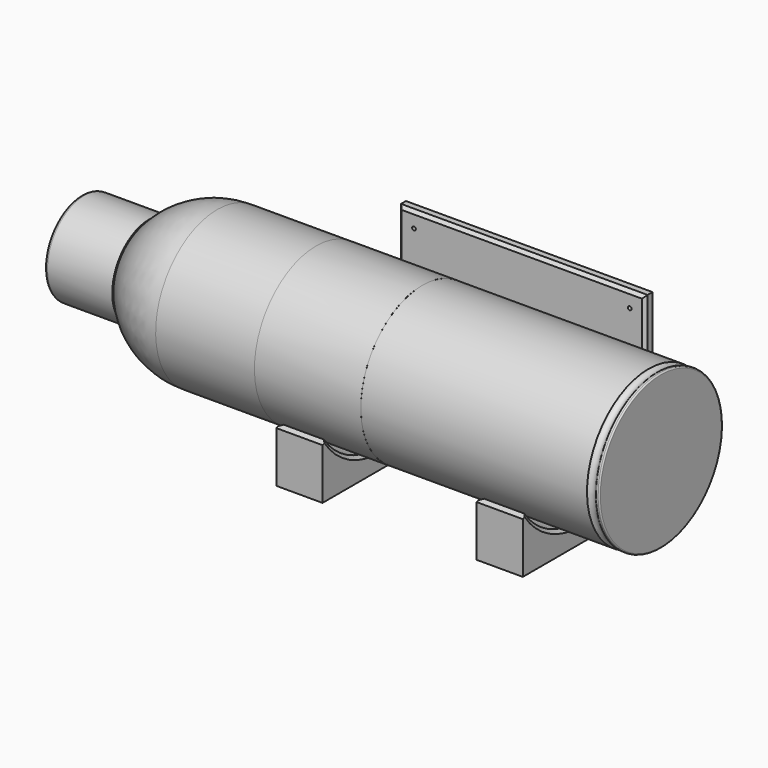
from build123d import *

# Parameters (mm, degrees)
F1_DEPTH     = 50.8
F2_T1_DEPTH  = 124.1425594427
F3_W         = 63.5
F3_H         = 53.3753879368
F4_DEPTH     = 25.4
F5_T1_DEPTH  = 63.5
F5_T3_DEPTH  = 108.1320747894
F5_T5_DEPTH  = 38.570501885
F5_T10_ANGLE = 111.4913949057
F5_T15_ANGLE = 111.4913949057
F5_T18_ANGLE = 150.4795795225
F5_T20_ANGLE = 150.4795795225
F5_T25_DEPTH = 64.906372973
F5_T29_ANGLE = 111.4913949057
F5_T36_ANGLE = 111.4913949057
F5_T40_DEPTH = 64.906372973
F6_R         = 0.762
F7_DEPTH     = 3.81
F10_W        = 5.08
F10_H        = 15.875
F14_R        = 2.54
F19_R        = 0.508
F20_R        = 1.3252507726
F21_DEPTH    = 25.4
F22_W        = 43.8366280696
F22_H        = 31.7754


# Not quite as in the source:
# - a fillet or chamfer that OpenCascade refuses, or shapes differently, is made with other operations: its cross-section is extruded or revolved along the edge and cut away or added
# - a pattern or mirror of a feature is missing from the dataset's text; its kind, count and spacing are read off the source's solid


with BuildPart() as f1:
    # F0 (on Right) → F1 (new body, symmetric)
    with BuildSketch(Plane.YZ):
        with BuildLine():
            Line((33.401, 35.3044644903), (33.401, 0))
            ThreePointArc((33.401, 0), (7.9787555162, -32.4340293737), (-29.58910577, -15.4955355097))
            Line((-29.58910577, -15.4955355097), (-29.58910577, -40.8955355097))
            Line((-29.58910577, -40.8955355097), (37.211, -40.8955355097))
            Line((37.211, -40.8955355097), (37.211, 35.3044644903))
            Line((37.211, 35.3044644903), (33.401, 35.3044644903))
        make_face()
    extrude(amount=F1_DEPTH, both=True)

    # F2: chamfer of 5.08 on 1 edges, made by hand

    # F2_s2 → F2_t1 (cut)
    with BuildSketch(Plane.YZ.offset(-62.0712797213)):
        with BuildLine():
            Line((-29.7828322597, -19.9998833533), (-27.1236395633, -19.1581562557))
            Line((-27.1236395633, -19.1581562557), (-27.0405449137, -19.0996939669))
            ThreePointArc((-27.0405449137, -19.0996939669), (-28.414686405, -17.3624778434), (-29.4991008855, -15.4484008009))
            Line((-29.4991008855, -15.4484008009), (-29.69070577, -15.4955355097))
            ThreePointArc((-29.69070577, -15.4955355097), (-29.69070577, -17.7477094315), (-29.8844322597, -19.9998833533))
            Line((-29.8844322597, -19.9998833533), (-29.7828322597, -19.9998833533))
        make_face()
    extrude(amount=F2_T1_DEPTH, mode=Mode.SUBTRACT)

    # F3 (on face) → F4 (cut)
    with BuildSketch(Plane(origin=(0, 0, -40.8955355097), x_dir=(1, 0, 0), z_dir=(0, 0, -1))):
        with Locations((0, 2.9014118016)):
            Rectangle(F3_W, F3_H)
    extrude(amount=-F4_DEPTH, mode=Mode.SUBTRACT)

    # F5: chamfer of 1.27 on 8 edges, made by hand

    # F5_s2 → F5_t1 (cut)
    with BuildSketch(Plane.YZ.offset(-31.75)):
        with BuildLine():
            Line((24.1384696333, -23.0859499429), (23.7862821668, -23.9637427164))
            Line((23.7862821668, -23.9637427164), (23.7862821668, -23.4486584196))
            ThreePointArc((23.7862821668, -23.4486584196), (23.9794328881, -23.2510988852), (24.1384696333, -23.0859499429))
        make_face()
    extrude(amount=F5_T1_DEPTH, mode=Mode.SUBTRACT)

    # F5_s4 → F5_t3 (cut)
    with BuildSketch(Plane.YZ.offset(-54.0660373947)):
        Polygon((34.671, 35.3044644903), (33.401, 34.0344644903), (33.401, 35.3044644903), align=None)
    extrude(amount=F5_T3_DEPTH, mode=Mode.SUBTRACT)

    # F5_s6 → F5_t5 (cut)
    with BuildSketch(Plane.XY):
        Polygon((-50.8, 34.671), (-49.53, 33.401), (-50.8, 33.401), align=None)
        Polygon((50.8, 34.671), (49.53, 33.401), (50.8, 33.401), align=None)
    extrude(amount=F5_T5_DEPTH, mode=Mode.SUBTRACT)


with BuildPart() as f5_tool8:
    # F5_s9 → F5_t10 (revolve)
    with BuildSketch(Plane(origin=(0, 0, 0), x_dir=(1, 0, 0), z_dir=(0, -0.4927798926, 0.8701539964))):
        Polygon((-33.02, -33.401), (-31.75, -34.671), (-31.75, -33.401), align=None)
    revolve(axis=Axis((-31.75, 0, 0), (1, 0, 0)), revolution_arc=F5_T10_ANGLE)

    split(bisect_by=Plane.XZ.offset(-23.7862821668), keep=Keep.TOP)


with BuildPart() as f1_1:
    add(f1.part)

    # F5_t7: cut F5_tool8
    add(f5_tool8.part, mode=Mode.SUBTRACT)


with BuildPart() as f5_tool13:
    # F5_s14 → F5_t15 (revolve)
    with BuildSketch(Plane(origin=(0, 0, 0), x_dir=(1, 0, 0), z_dir=(0, -0.4927798926, 0.8701539964))):
        Polygon((33.02, -33.401), (31.75, -34.671), (31.75, -33.401), align=None)
    revolve(axis=Axis((31.75, 0, 0), (1, 0, 0)), revolution_arc=F5_T15_ANGLE)

    split(bisect_by=Plane.XZ.offset(-23.7862821668), keep=Keep.TOP)


with BuildPart() as f1_2:
    add(f1_1.part)

    # F5_t12: cut F5_tool13
    add(f5_tool13.part, mode=Mode.SUBTRACT)

    # F5_s17 → F5_t18 (revolve, cut)
    with BuildSketch(Plane.XY):
        Polygon((50.8, 34.671), (49.53, 33.401), (50.8, 33.401), align=None)
    revolve(axis=Axis((50.8, 0, 0), (-1, 0, 0)), revolution_arc=F5_T18_ANGLE, mode=Mode.SUBTRACT)

    # F5_s19 → F5_t20 (revolve, cut)
    with BuildSketch(Plane.XY):
        Polygon((-50.8, 34.671), (-49.53, 33.401), (-50.8, 33.401), align=None)
    revolve(axis=Axis((-50.8, 0, 0), (-1, 0, 0)), revolution_arc=F5_T20_ANGLE, mode=Mode.SUBTRACT)


with BuildPart() as f5_tool23:
    # F5_s24 → F5_t25 (new body)
    with BuildSketch(Plane.YZ.offset(-33.156372973)):
        with BuildLine():
            Line((24.1384696333, -23.0859499429), (23.7862821668, -23.9637427164))
            Line((23.7862821668, -23.9637427164), (23.7862821668, -23.4486584196))
            ThreePointArc((23.7862821668, -23.4486584196), (23.9794328881, -23.2510988852), (24.1384696333, -23.0859499429))
        make_face()
    extrude(amount=F5_T25_DEPTH)

    split(bisect_by=Plane.YZ.offset(-31.75), keep=Keep.BOTTOM)


with BuildPart() as f5_tool27:
    # F5_s28 → F5_t29 (revolve)
    with BuildSketch(Plane(origin=(0, 0, 0), x_dir=(1, 0, 0), z_dir=(0, -0.4927798926, 0.8701539964))):
        Polygon((-33.02, -33.401), (-31.75, -34.671), (-31.75, -33.401), align=None)
    revolve(axis=Axis((-31.75, 0, 0), (1, 0, 0)), revolution_arc=F5_T29_ANGLE)

    split(bisect_by=Plane.XZ.offset(-23.7862821668), keep=Keep.BOTTOM)


with BuildPart() as f5_tool23_1:
    add(f5_tool23.part)

    # F5_t31: intersect F5_tool27
    add(f5_tool27.part, mode=Mode.INTERSECT)


with BuildPart() as f1_3:
    add(f1_2.part)

    # F5_t21: cut F5_tool23
    add(f5_tool23_1.part, mode=Mode.SUBTRACT)


with BuildPart() as f5_tool34:
    # F5_s35 → F5_t36 (revolve)
    with BuildSketch(Plane(origin=(0, 0, 0), x_dir=(1, 0, 0), z_dir=(0, -0.4927798926, 0.8701539964))):
        Polygon((33.02, -33.401), (31.75, -34.671), (31.75, -33.401), align=None)
    revolve(axis=Axis((31.75, 0, 0), (1, 0, 0)), revolution_arc=F5_T36_ANGLE)

    split(bisect_by=Plane.XZ.offset(-23.7862821668), keep=Keep.BOTTOM)


with BuildPart() as f5_tool38:
    # F5_s39 → F5_t40 (new body)
    with BuildSketch(Plane.YZ.offset(-31.75)):
        with BuildLine():
            Line((24.1384696333, -23.0859499429), (23.7862821668, -23.9637427164))
            Line((23.7862821668, -23.9637427164), (23.7862821668, -23.4486584196))
            ThreePointArc((23.7862821668, -23.4486584196), (23.9794328881, -23.2510988852), (24.1384696333, -23.0859499429))
        make_face()
    extrude(amount=F5_T40_DEPTH)

    split(bisect_by=Plane.YZ.offset(31.75), keep=Keep.TOP)


with BuildPart() as f5_tool34_1:
    add(f5_tool34.part)

    # F5_t42: intersect F5_tool38
    add(f5_tool38.part, mode=Mode.INTERSECT)


with BuildPart() as f1_4:
    add(f1_3.part)

    # F5_t32: cut F5_tool34
    add(f5_tool34_1.part, mode=Mode.SUBTRACT)

    # F6 (on face) → F7 (cut, through all)
    with BuildSketch(Plane(origin=(0, 37.211, 0), x_dir=(-1, 0, 0), z_dir=(0, 1, 0))):
        with Locations((-44.45, 28.9544644903)):
            Circle(F6_R)
    f7 = extrude(amount=-F7_DEPTH, mode=Mode.SUBTRACT)

    # F7_copies: F7 across plane
    add(f7.mirror(Plane(origin=(0, 0, 0), x_dir=(0, 0, -1), z_dir=(-1, 0, 0))), mode=Mode.SUBTRACT)


with BuildPart() as f9:
    # F8 (on Front) → F9 (revolve)
    with BuildSketch(Plane.XZ):
        with BuildLine():
            Line((-133.4317177534, 0), (78.9947096897, 0))
            Line((78.9947096897, 0), (78.9947096897, 31.75))
            Line((78.9947096897, 31.75), (-98.8052903103, 31.75))
            ThreePointArc((-98.8052903103, 31.75), (-120.222127041, 24.7786799307), (-133.4317177534, 6.5362318419))
            Line((-133.4317177534, 6.5362318419), (-133.4317177534, 0))
        make_face()
    revolve(axis=Axis((-27.2185040319, 0, 0), (-1, 0, 0)))


with BuildPart() as f11:
    # F10 (on Front) → F11 (revolve)
    with BuildSketch(Plane.XZ):
        with Locations((-131.9004494365, 7.9375)):
            Rectangle(F10_W, F10_H)
    revolve(axis=Axis((-131.9004494365, 0, 0), (-1, 0, 0)))

    # F14
    f14_edges = [f11.edges().sort_by_distance(p)[0] for p in [
        (-134.440449, 0, -15.875),
    ]]
    fillet(f14_edges, radius=F14_R)


with BuildPart() as f13:
    # F12 (on Front) → F13 (revolve)
    with BuildSketch(Plane.XZ):
        Polygon((-138.9863938093, 0), (-134.2986822128, 0), (-134.2986822128, 11.3506736234), (-138.9863938093, 11.3506736234), (-138.9863938093, 7.7716847882), (-149.6194899082, 7.7716847882), (-149.6194899082, 0), align=None)
    revolve(axis=Axis((-144.3029418588, 0, 0), (1, 0, 0)))

    # F20 (on Front) → F21 (cut)
    with BuildSketch(Plane.XZ):
        with Locations((-147.1612453461, 0)):
            Circle(F20_R)
    extrude(amount=F21_DEPTH, mode=Mode.SUBTRACT)


with BuildPart() as f16:
    # F15 (on Front) → F16 (revolve)
    with BuildSketch(Plane.XZ):
        with BuildLine():
            Line((-154.7955721617, 17.78), (-154.7955721617, 0))
            Line((-154.7955721617, 0), (-153.5255721617, 0))
            Line((-153.5255721617, 0), (-153.5255721617, 16.51))
            ThreePointArc((-153.5255721617, 16.51), (-153.1535977738, 17.4080256121), (-152.2555721617, 17.78))
            Line((-152.2555721617, 17.78), (-126.8555721617, 17.78))
            Line((-126.8555721617, 17.78), (-126.8555721617, 19.05))
            Line((-126.8555721617, 19.05), (-153.5255721617, 19.05))
            ThreePointArc((-153.5255721617, 19.05), (-154.4235977738, 18.6780256121), (-154.7955721617, 17.78))
        make_face()
    revolve(axis=Axis((-154.1605721617, 0, 0), (1, 0, 0)))


with BuildPart() as f18:
    # F17 (on Front) → F18 (revolve)
    with BuildSketch(Plane.XZ):
        with BuildLine():
            Line((78.9947096897, 31.75), (78.9947096897, 0))
            Line((78.9947096897, 0), (84.0747096897, 0))
            Line((84.0747096897, 0), (84.0747096897, 31.75))
            Line((84.0747096897, 31.75), (82.6066508889, 31.75))
            ThreePointArc((82.6066508889, 31.75), (80.8006802893, 30.7873346522), (78.9947096897, 31.75))
        make_face()
    revolve(axis=Axis((81.5347096897, 0, 0), (1, 0, 0)))

    # F19
    f19_edges = [f18.edges().sort_by_distance(p)[0] for p in [
        (82.606651, 0, -31.75),
        (84.07471, 0, -31.75),
    ]]
    fillet(f19_edges, radius=F19_R)


with BuildPart() as f23:
    # F22 (on Front) → F23 (revolve)
    with BuildSketch(Plane.XZ):
        with Locations((-36.1483705929, 15.8877)):
            Rectangle(F22_W, F22_H)
    revolve(axis=Axis((-36.1483705929, 0, 0), (1, 0, 0)))


solid = Compound([f1_4.part, f9.part, f11.part, f13.part, f16.part, f18.part, f23.part])
